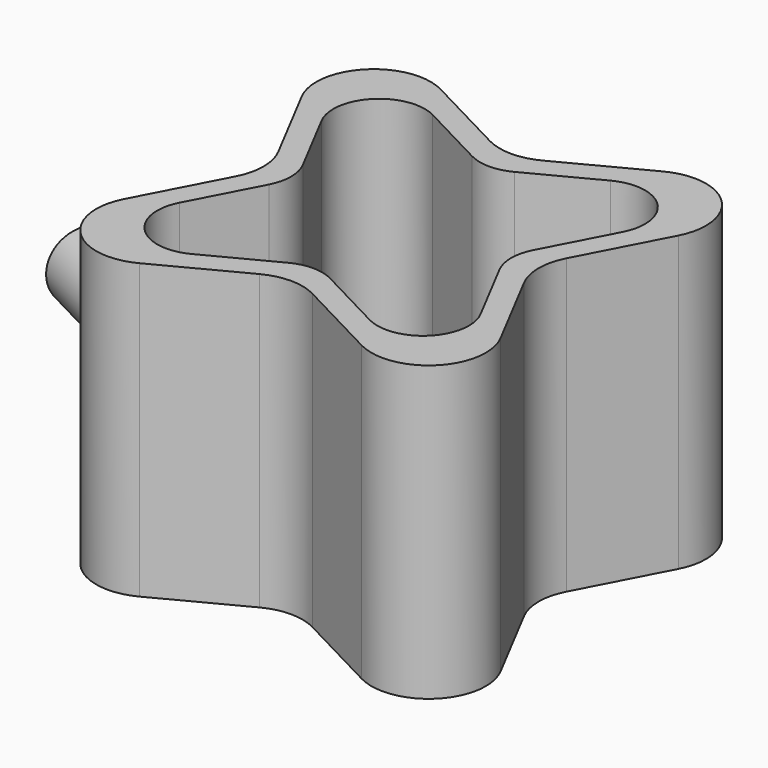
from build123d import *

# Parameters (mm, degrees)
F1_DEPTH = 203.2
F2_R     = 24.4501828069
F3_DEPTH = 127


# Not quite as in the source:
# - ends of sketch curves that miss each other by under 0.0002 mm in the source are joined
# - the program builds the solid bodies; features that only make, move or delete a surface that nothing else refers to are left out


with BuildPart() as f1:
    # F0 (on Top) → F1 (new body)
    with BuildSketch(Plane.XY):
        with BuildLine():
            Line((-18.3351678, 99.7503212), (-76.9148068, 130.3502854))
            ThreePointArc((-76.9148068, 130.3502854), (-123.2518754265, 123.2518754265), (-130.3502933453, 76.9148026497))
            Line((-130.3502933453, 76.9148026497), (-99.7503212, 18.3351678))
            ThreePointArc((-99.7503212, 18.3351678), (-95.25, -1.12567e-05), (-99.7503332097, -18.3351869265))
            Line((-99.7503332097, -18.3351869265), (-130.3502854, -76.9148322))
            ThreePointArc((-130.3502854, -76.9148322), (-123.2518716246, -123.2518792283), (-76.9148130735, -130.3502987903))
            Line((-76.9148130735, -130.3502987903), (-18.3351678, -99.7503466))
            ThreePointArc((-18.3351678, -99.7503466), (1.12567e-05, -95.2500254), (18.3351869265, -99.7503586097))
            Line((18.3351869265, -99.7503586097), (76.9148322, -130.3503108))
            ThreePointArc((76.9148322, -130.3503108), (123.2518754265, -123.2518754265), (130.3503092141, -76.9148330284))
            Line((130.3503092141, -76.9148330284), (99.7503466, -18.3351932))
            ThreePointArc((99.7503466, -18.3351932), (95.25, -1.12567e-05), (99.7503282309, 18.3351773954))
            Line((99.7503282309, 18.3351773954), (130.3503108, 76.9148068))
            ThreePointArc((130.3503108, 76.9148068), (123.2518792283, 123.2518716246), (76.9148226046, 130.3503037691))
            Line((76.9148226046, 130.3503037691), (18.3351932, 99.7503212))
            ThreePointArc((18.3351932, 99.7503212), (1.12567e-05, 95.25), (-18.3351678, 99.7503212))
        make_face()
        with BuildLine():
            ThreePointArc((-104.2802295109, 61.5318322315), (-98.6015083009, 98.6014923815), (-61.5318521865, 104.2802399347))
            Line((-61.5318521865, 104.2802399347), (-14.6681444, 79.8002468))
            ThreePointArc((-14.6681444, 79.8002468), (0, 76.2), (14.6681373897, 79.8002602202))
            Line((14.6681373897, 79.8002602202), (61.5318556, 104.2802334))
            ThreePointArc((61.5318556, 104.2802334), (98.601504143, 98.6014965393), (104.280234956, 61.5318426553))
            Line((104.280234956, 61.5318426553), (79.8002722, 14.6681444))
            ThreePointArc((79.8002722, 14.6681444), (76.2, -1.12567e-05), (79.8002760891, -14.6681677685))
            Line((79.8002760891, -14.6681677685), (104.2802588, -61.5318556))
            ThreePointArc((104.2802588, -61.5318556), (98.6015003412, -98.6015003412), (61.5318626103, -104.2802453798))
            Line((61.5318626103, -104.2802453798), (14.6681444, -79.8002722))
            ThreePointArc((14.6681444, -79.8002722), (0, -76.2000254), (-14.6681373897, -79.8002856202))
            Line((-14.6681373897, -79.8002856202), (-61.5318556, -104.2802588))
            ThreePointArc((-61.5318556, -104.2802588), (-98.6015044991, -98.6014961833), (-104.2802399347, -61.5318521865))
            Line((-104.2802399347, -61.5318521865), (-79.8002468, -14.6681698))
            ThreePointArc((-79.8002468, -14.6681698), (-76.2, -1.12567e-05), (-79.8002602202, 14.6681373897))
            Line((-79.8002602202, 14.6681373897), (-104.2802295109, 61.5318322315))
        make_face(mode=Mode.SUBTRACT)
    extrude(amount=F1_DEPTH)

    # F2 (on face) → F3 (join)
    with BuildSketch(Plane(origin=(-70.8422549592, 37.0055279036, 0), x_dir=(-0.4630021293, -0.8863571674, 0), z_dir=(-0.8863571674, 0.4630021293, 0))):
        with Locations((94.1798388958, 94.7972759604)):
            Circle(F2_R)
    extrude(amount=F3_DEPTH)


solid = f1.part
